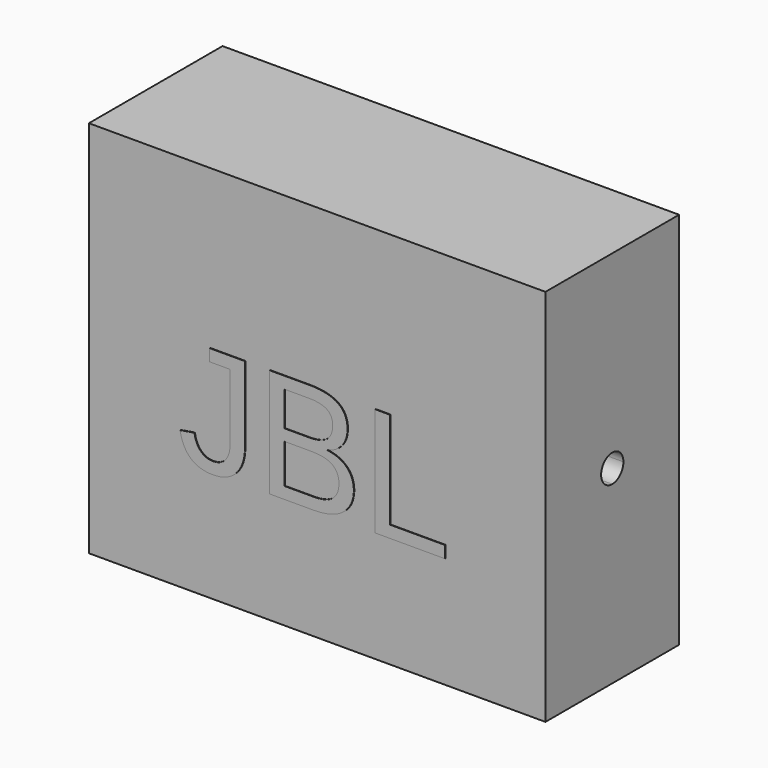
from build123d import *

# Parameters (mm, degrees)
F0_W         = 82
F0_H         = 68
F1_DEPTH     = 30
F2_TEXT_SIZE = 28.4191829485
F3_DEPTH     = 0.1
F5_DEPTH     = 10


# Not quite as in the source:
# - Text() gives the source's letters only with a copy of the font that has no kerning and outlines rounded to 1/6400 em; it was checked with that copy


with BuildPart() as f1:
    # F0 (on Front) → F1 (new body)
    with BuildSketch(Plane.XZ):
        with Locations((0, 38)):
            Rectangle(F0_W, F0_H)
    extrude(amount=F1_DEPTH)

    # F4 (on face) → F5 (cut)
    with BuildSketch(Plane.YZ.offset(41)):
        with BuildLine():
            Line((-15, 38), (-12.5, 38))
            ThreePointArc((-12.5, 38), (-13.232233047, 39.767766953), (-15, 40.5))
            Line((-15, 40.5), (-15, 38))
        make_face()
        with BuildLine():
            ThreePointArc((-15, 35.5), (-13.232233047, 36.232233047), (-12.5, 38))
            Line((-12.5, 38), (-15, 38))
            Line((-15, 38), (-15, 35.5))
        make_face()
        with BuildLine():
            Line((-15, 38), (-15, 40.5))
            ThreePointArc((-15, 40.5), (-16.767766953, 39.767766953), (-17.5, 38))
            Line((-17.5, 38), (-15, 38))
        make_face()
        with BuildLine():
            ThreePointArc((-17.5, 38), (-16.767766953, 36.232233047), (-15, 35.5))
            Line((-15, 35.5), (-15, 38))
            Line((-15, 38), (-17.5, 38))
        make_face()
    extrude(amount=-F5_DEPTH, mode=Mode.SUBTRACT)


with BuildPart() as f3:
    # F2 (on face) → F3 (new body)
    with BuildSketch(Plane.XZ.offset(30)):
        with Locations((-25, 24)):
            Text('JBL', F2_TEXT_SIZE, font='Arimo', text_align=(TextAlign.LEFT, TextAlign.BOTTOM))
    extrude(amount=F3_DEPTH)


solid = Compound([f1.part, f3.part])
